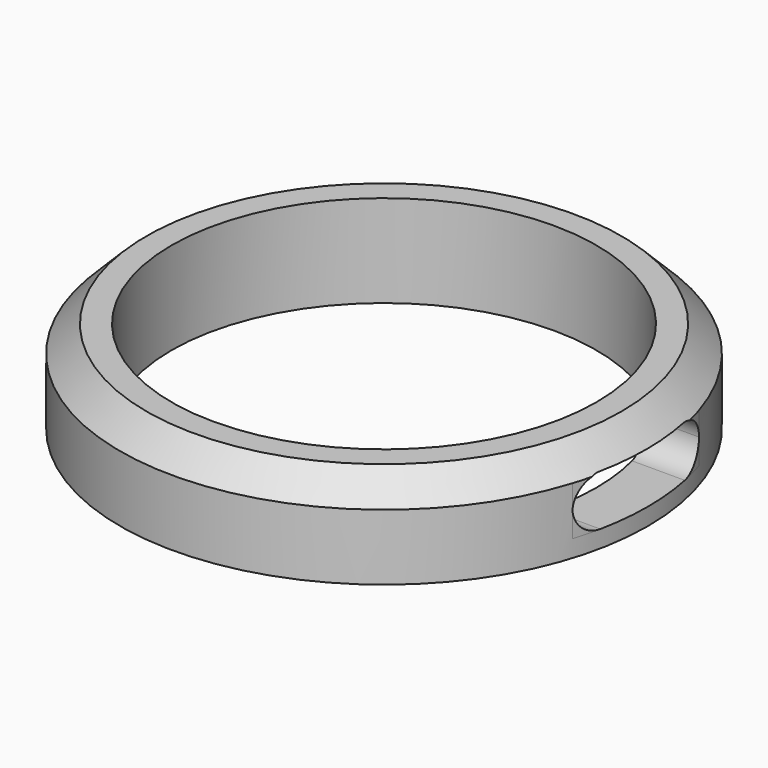
from build123d import *

# Parameters (mm, degrees)
F0_R         = 10
F0_R_2       = 8.05
F1_DEPTH     = 3.5
F3_DEPTH     = 16.9
F4_T4_DEPTH  = 7.0692849199
F4_S5_R      = 10
F4_T6_DEPTH  = 5
F4_S7_R      = 8.05
F4_T8_DEPTH  = 5
F4_T12_DEPTH = 7.0692849199
F4_S13_R     = 10
F4_T14_DEPTH = 5
F4_S15_R     = 8.05
F4_T16_DEPTH = 5
F4_T20_DEPTH = 7.0692849199
F4_S21_R     = 10
F4_T22_DEPTH = 5
F4_S23_R     = 8.05
F4_T24_DEPTH = 5
F4_T28_DEPTH = 7.0692849199
F4_S29_R     = 10
F4_T30_DEPTH = 5
F4_S31_R     = 8.05
F4_T32_DEPTH = 5


# Not quite as in the source:
# - a fillet or chamfer that OpenCascade refuses, or shapes differently, is made with other operations: its cross-section is extruded or revolved along the edge and cut away or added


with BuildPart() as f1:
    # F0 (on Top) → F1 (new body)
    with BuildSketch(Plane.XY):
        Circle(F0_R)
        Circle(F0_R_2, mode=Mode.SUBTRACT)
    extrude(amount=F1_DEPTH)

    # F2 (on Right) → F3 (cut)
    with BuildSketch(Plane.YZ):
        Polygon((3, 0.65), (3, 2.55), (-3, 2.55), (-3, 0.65), (0, 0.65), align=None)
    extrude(amount=F3_DEPTH, mode=Mode.SUBTRACT)

    # F4: fillet of radius 1 on 4 edges, made by hand


with BuildPart() as f4_tool2:
    # F4_s3 → F4_t4 (new body)
    with BuildSketch(Plane.YZ.offset(4.9701070943)):
        with BuildLine():
            ThreePointArc((2, 2.55), (2.7071067812, 2.2571067812), (3, 1.55))
            Line((3, 1.55), (3, 2.55))
            Line((3, 2.55), (2, 2.55))
        make_face()
    extrude(amount=F4_T4_DEPTH)

    # F4_s5 → F4_t6 (intersect, symmetric)
    with BuildSketch(Plane.XY.offset(2)):
        Circle(F4_S5_R)
    extrude(amount=F4_T6_DEPTH, both=True, mode=Mode.INTERSECT)

    # F4_s7 → F4_t8 (cut, symmetric)
    with BuildSketch(Plane.XY.offset(2)):
        Circle(F4_S7_R)
    extrude(amount=F4_T8_DEPTH, both=True, mode=Mode.SUBTRACT)


with BuildPart() as f1_1:
    add(f1.part)

    # F4_t1: union F4_tool2
    add(f4_tool2.part)


with BuildPart() as f4_tool10:
    # F4_s11 → F4_t12 (new body)
    with BuildSketch(Plane.YZ.offset(4.9701070943)):
        with BuildLine():
            ThreePointArc((2, 0.65), (2.7071067812, 0.9428932188), (3, 1.65))
            Line((3, 1.65), (3, 0.65))
            Line((3, 0.65), (2, 0.65))
        make_face()
    extrude(amount=F4_T12_DEPTH)

    # F4_s13 → F4_t14 (intersect, symmetric)
    with BuildSketch(Plane.XY.offset(1.1)):
        Circle(F4_S13_R)
    extrude(amount=F4_T14_DEPTH, both=True, mode=Mode.INTERSECT)

    # F4_s15 → F4_t16 (cut, symmetric)
    with BuildSketch(Plane.XY.offset(1.1)):
        Circle(F4_S15_R)
    extrude(amount=F4_T16_DEPTH, both=True, mode=Mode.SUBTRACT)


with BuildPart() as f1_2:
    add(f1_1.part)

    # F4_t9: union F4_tool10
    add(f4_tool10.part)


with BuildPart() as f4_tool18:
    # F4_s19 → F4_t20 (new body)
    with BuildSketch(Plane.YZ.offset(4.9701070943)):
        with BuildLine():
            ThreePointArc((-3, 1.55), (-2.7071067812, 2.2571067812), (-2, 2.55))
            Line((-2, 2.55), (-3, 2.55))
            Line((-3, 2.55), (-3, 1.55))
        make_face()
    extrude(amount=F4_T20_DEPTH)

    # F4_s21 → F4_t22 (intersect, symmetric)
    with BuildSketch(Plane.XY.offset(2)):
        Circle(F4_S21_R)
    extrude(amount=F4_T22_DEPTH, both=True, mode=Mode.INTERSECT)

    # F4_s23 → F4_t24 (cut, symmetric)
    with BuildSketch(Plane.XY.offset(2)):
        Circle(F4_S23_R)
    extrude(amount=F4_T24_DEPTH, both=True, mode=Mode.SUBTRACT)


with BuildPart() as f1_3:
    add(f1_2.part)

    # F4_t17: union F4_tool18
    add(f4_tool18.part)


with BuildPart() as f4_tool26:
    # F4_s27 → F4_t28 (new body)
    with BuildSketch(Plane.YZ.offset(4.9701070943)):
        with BuildLine():
            ThreePointArc((-2, 0.65), (-2.7071067812, 0.9428932188), (-3, 1.65))
            Line((-3, 1.65), (-3, 0.65))
            Line((-3, 0.65), (-2, 0.65))
        make_face()
    extrude(amount=F4_T28_DEPTH)

    # F4_s29 → F4_t30 (intersect, symmetric)
    with BuildSketch(Plane.XY.offset(1.1)):
        Circle(F4_S29_R)
    extrude(amount=F4_T30_DEPTH, both=True, mode=Mode.INTERSECT)

    # F4_s31 → F4_t32 (cut, symmetric)
    with BuildSketch(Plane.XY.offset(1.1)):
        Circle(F4_S31_R)
    extrude(amount=F4_T32_DEPTH, both=True, mode=Mode.SUBTRACT)


with BuildPart() as f1_4:
    add(f1_3.part)

    # F4_t25: union F4_tool26
    add(f4_tool26.part)

    # F5: chamfer of 1 on 1 edges, made by hand

    # F5_s1 → F5_t2 (revolve, cut)
    with BuildSketch(Plane.XZ):
        Polygon((10, 2.5), (9, 3.5), (10, 3.5), align=None)
    revolve(axis=Axis((0, 0, 3.5), (0, 0, 1)), mode=Mode.SUBTRACT)


solid = f1_4.part
